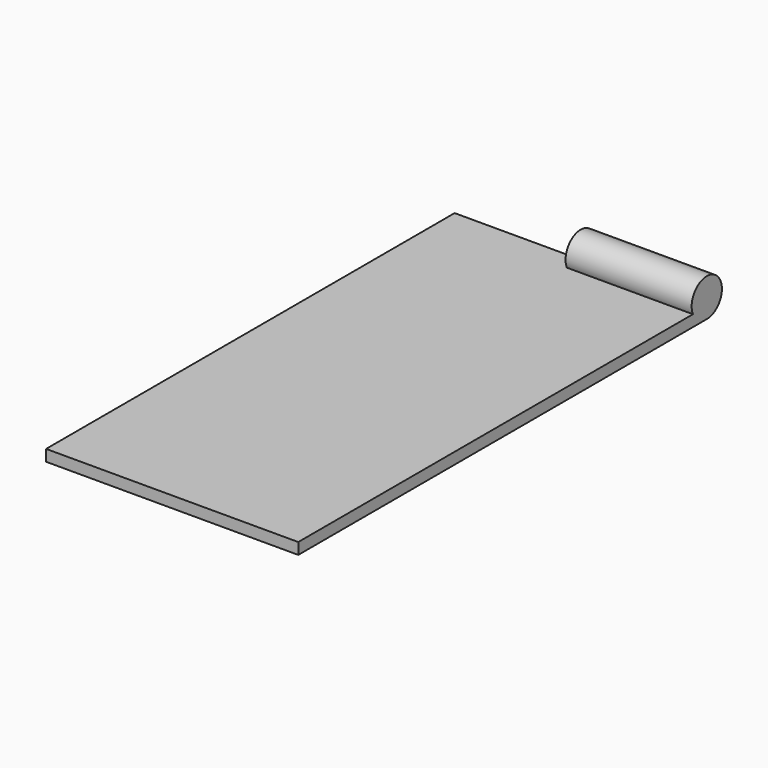
from build123d import *

# Parameters (mm, degrees)
F0_W     = 40
F0_H     = 81
F1_DEPTH = 1.8
F3_DEPTH = 20


with BuildPart() as f1:
    # F0 (on Top) → F1 (new body)
    with BuildSketch(Plane.XY):
        with Locations((20, -40.5)):
            Rectangle(F0_W, F0_H)
    extrude(amount=F1_DEPTH)

    # F2 (on face) → F3 (join)
    with BuildSketch(Plane.YZ.offset(40)):
        with BuildLine():
            Line((0, 1.8), (0, 0))
            ThreePointArc((0, 0), (2.1213203436, 0.8786796564), (3, 3))
            ThreePointArc((3, 3), (-0.6129289311, 5.9367189388), (-2.749545417, 1.8))
            Line((-2.749545417, 1.8), (0, 1.8))
        make_face()
        with BuildLine():
            ThreePointArc((-2.749545417, 1.8), (-1.6431676725, 0.4900199204), (0, 0))
            Line((0, 0), (0, 1.8))
            Line((0, 1.8), (-2.749545417, 1.8))
        make_face()
    extrude(amount=-F3_DEPTH)


solid = f1.part
